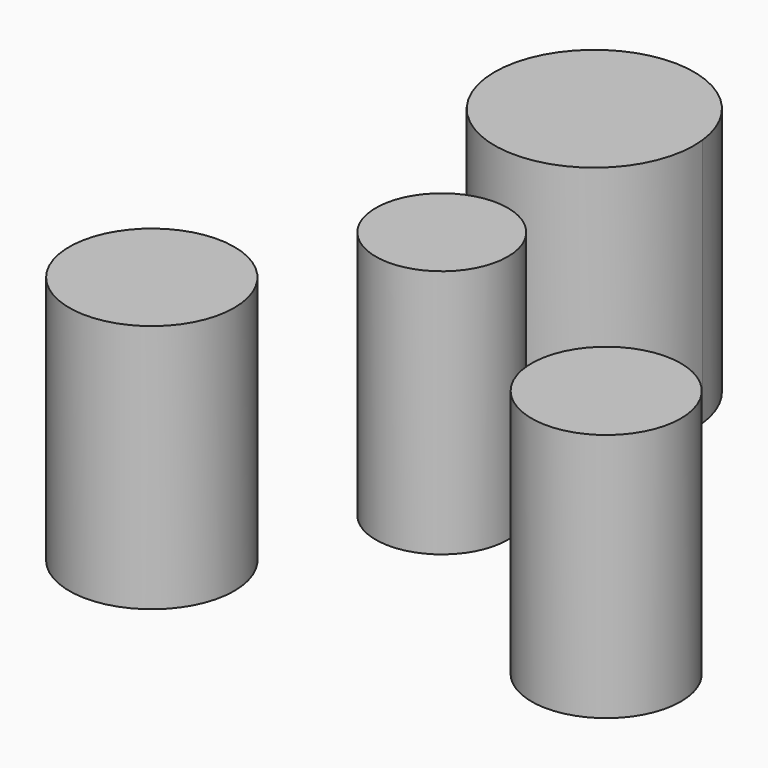
from build123d import *

# Parameters (mm, degrees)
F5_DEPTH = 25.4
F4_R     = 6.7259983567
F1_R     = 8.4107438271
F2_R     = 7.608509741


# Not quite as in the source:
# - the program builds the solid bodies; features that only make, move or delete a surface that nothing else refers to are left out


with BuildPart() as f5:
    # F0 (on Top) → F5 (new body)
    with BuildSketch(Plane.XY):
        with BuildLine():
            ThreePointArc((-11.4537579939, 7.812615484), (0.3902658063, 1.0605246734), (8.2872472703, 12.1739991009))
            ThreePointArc((8.2872472703, 12.1739991009), (4.5861760116, 18.8798650483), (-2.7458775352, 21.0951657847))
            ThreePointArc((-2.7458775352, 21.0951657847), (-10.2972299306, 16.5500756507), (-11.4537579939, 7.812615484))
        make_face()
    extrude(amount=F5_DEPTH)


with BuildPart() as f5b:
    # F4 (on Top) → F5, piece 2 (new body)
    with BuildSketch(Plane.XY):
        with Locations((2.0192693919, -13.2251810282)):
            Circle(F4_R)
    extrude(amount=F5_DEPTH)


with BuildPart() as f5c:
    # F1 (on Top) → F5, piece 3 (new body)
    with BuildSketch(Plane.XY):
        with Locations((-11.1536812037, -33.7025821209)):
            Circle(F1_R)
    extrude(amount=F5_DEPTH)


with BuildPart() as f5d:
    # F2 (on Top) → F5, piece 4 (new body)
    with BuildSketch(Plane.XY):
        with Locations((29.3082781136, -26.3951309025)):
            Circle(F2_R)
    extrude(amount=F5_DEPTH)


solid = Compound([f5.part, f5b.part, f5c.part, f5d.part])
